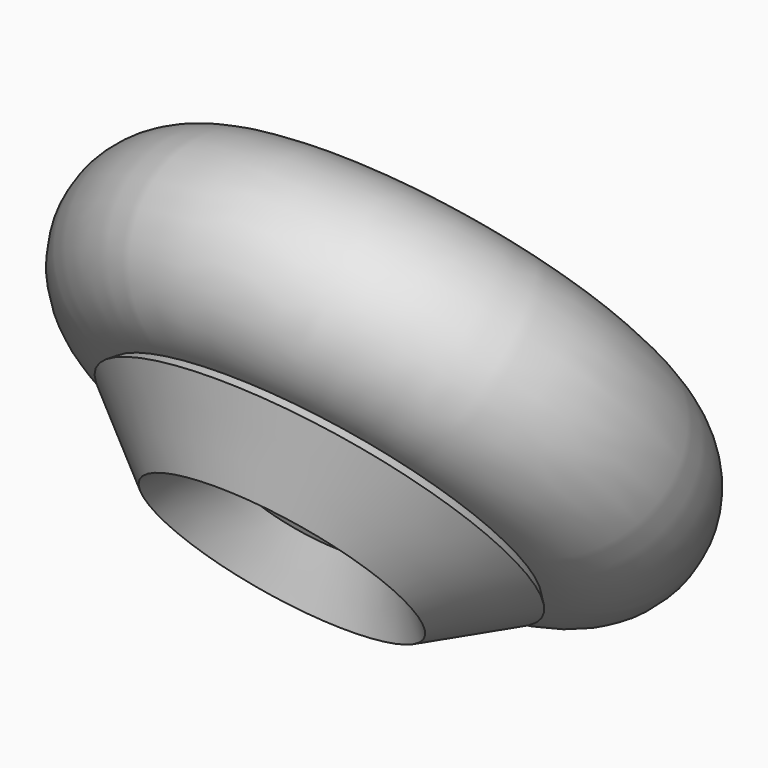
from build123d import *


# Not quite as in the source:
# - a feature names something its author has since deleted; it is built from what else it names


with BuildPart() as f1:
    # F0 (on Top) → F1 (revolve)
    with BuildSketch(Plane.XY):
        with BuildLine():
            ThreePointArc((-126.2936090108, -60.9435376982), (-125.5275482396, -14.8005998046), (-79.8075346727, -8.5206375433))
            ThreePointArc((-79.8075346727, -8.5206375433), (-158.7697402428, 14.6769568368), (-126.2936090108, -60.9435376982))
        make_face()
    revolve(axis=Axis((-29.3286815286, -4.3713711202, 0), (0.6373696425, -0.7705581995, 0)))


with BuildPart() as f1b:
    # F0 (on Top) → F1, piece 2 (revolve)
    with BuildSketch(Plane.XY):
        with BuildLine():
            ThreePointArc((-79.8075346727, -8.5206375433), (-79.4042868466, -11.9972450764), (-79.2696049846, -15.4945682734))
            ThreePointArc((-79.2696049846, -15.4945682734), (-93.1413013496, -48.1934435463), (-126.2936090108, -60.9435376982))
            ThreePointArc((-126.2936090108, -60.9435376982), (-86.9802869652, -71.6637251276), (-63.5586823019, -38.3187383413))
            ThreePointArc((-63.5586823019, -38.3187383413), (-67.8848955276, -21.3485290428), (-79.8075346727, -8.5206375433))
        make_face()
    revolve(axis=Axis((-29.3286815286, -4.3713711202, 0), (0.6373696425, -0.7705581995, 0)))


with BuildPart() as f3:
    # F2 (on Right) → F3 (revolve)
    with BuildSketch(Plane.YZ):
        with BuildLine():
            ThreePointArc((-337.8788083792, 218.5828652107), (-297.7077005564, 216.6281105112), (-258.2443356514, 224.3858034685))
            ThreePointArc((-258.2443356514, 224.3858034685), (-175.3359519396, 284.7466982936), (-143.6770656998, 382.2913169861))
            ThreePointArc((-143.6770656998, 382.2913169861), (-363.9074469759, 539.3269656823), (-440.6045777253, 279.9446880817))
            Line((-440.6045777253, 279.9446880817), (-337.8788083792, 279.9446880817))
            Line((-337.8788083792, 279.9446880817), (-337.8788083792, 218.5828652107))
        make_face()
    revolve(axis=Axis((0, -155.7009387761, 93.5366116464), (0, -0.7616262804, -0.6480165191)))


with BuildPart() as f3b:
    # F2 (on Right) → F3, piece 2 (revolve)
    with BuildSketch(Plane.YZ):
        with BuildLine():
            Line((-337.8788083792, 118.8967078924), (-337.8788083792, 178.4088192023))
            Line((-337.8788083792, 178.4088192023), (-337.8788083792, 218.5828652107))
            ThreePointArc((-337.8788083792, 218.5828652107), (-394.9590675899, 239.6923253669), (-440.6045777253, 279.9446880817))
            Line((-440.6045777253, 279.9446880817), (-458.6133658886, 279.9446880817))
            Line((-458.6133658886, 279.9446880817), (-458.6133658886, 118.8967078924))
            Line((-458.6133658886, 118.8967078924), (-337.8788083792, 118.8967078924))
        make_face()
        Polygon((-178.6098629236, 86.45485067), (-178.6098629236, 178.4088192023), (-258.2443356514, 224.3858034685), (-337.8788083792, 178.4088192023), (-337.8788083792, 118.8967078924), (-337.8788083792, 86.45485067), (-258.2443356514, 40.4778664038), align=None)
    revolve(axis=Axis((0, -155.7009387761, 93.5366116464), (0, -0.7616262804, -0.6480165191)))


solid = Compound([f1.part, f1b.part, f3.part, f3b.part])
